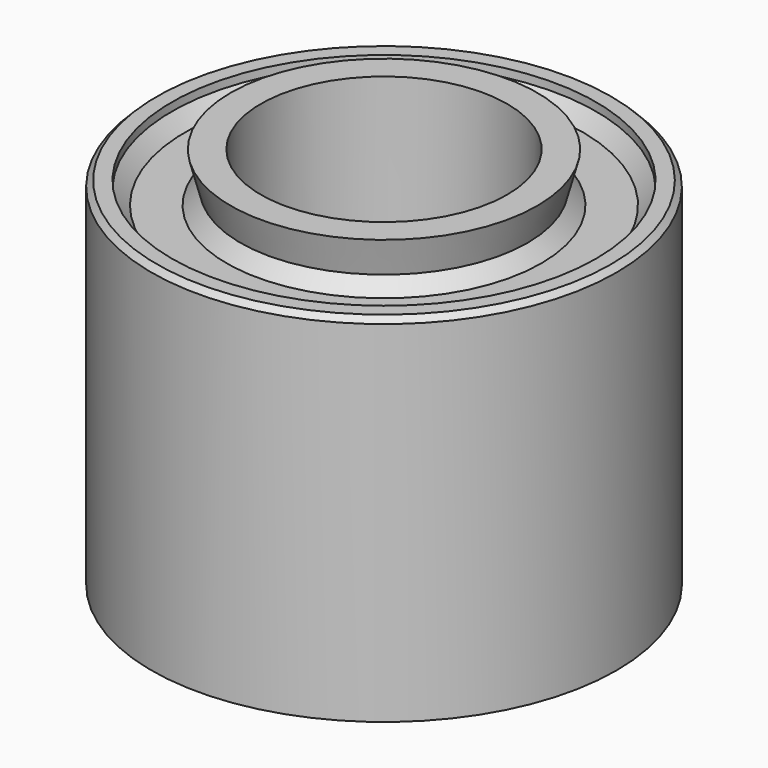
from build123d import *

# Parameters (mm, degrees)
F0_R      = 8.5
F1_DEPTH  = 13
F2_R      = 2.75
F3_DEPTH  = 13.001
F4_R      = 4.5
F5_DEPTH  = 10
F6_SIZE   = 0.2
F7_R      = 7.75
F7_R_2    = 5.25
F8_DEPTH  = 0.8
F9_DEPTH  = 1
F10_R     = 5.6
F10_R_2   = 4.5
F11_DEPTH = 1.5
F11_TAPER = 15


# Not quite as in the source:
# - a fillet or chamfer that OpenCascade refuses, or shapes differently, is made with other operations: its cross-section is extruded or revolved along the edge and cut away or added
# - a feature names something its author has since deleted; it is built from what else it names


with BuildPart() as f1:
    # F0 (on Top) → F1 (new body)
    with BuildSketch(Plane.XY):
        Circle(F0_R)
    extrude(amount=F1_DEPTH)

    # F2 (on face) → F3 (cut, through all)
    with BuildSketch(Plane.XY.offset(13)):
        Circle(F2_R)
    extrude(amount=-F3_DEPTH, mode=Mode.SUBTRACT)

    # F4 (on face) → F5 (cut)
    with BuildSketch(Plane.XY.offset(13)):
        Circle(F4_R)
    extrude(amount=-F5_DEPTH, mode=Mode.SUBTRACT)

    # F6
    f6_edges = [f1.edges().sort_by_distance(p)[0] for p in [
        (-8.5, 0, 13),
    ]]
    chamfer(f6_edges, length=F6_SIZE)

    # F7 (on face) → F8 (cut)
    with BuildSketch(Plane.XY.offset(13)):
        Circle(F7_R)
        Circle(F7_R_2, mode=Mode.SUBTRACT)
    extrude(amount=-F8_DEPTH, mode=Mode.SUBTRACT)

    # F9 (add): a face of the model
    f9_faces = [f1.faces().sort_by_distance(p)[0] for p in [
        (-5.101507576, 0, 13),
    ]]
    extrude(f9_faces, amount=F9_DEPTH)

    # F10 (on face) → F11 (join)
    with BuildSketch(Plane.XY.offset(14)):
        Circle(F10_R)
        Circle(F10_R_2, mode=Mode.SUBTRACT)
    extrude(amount=-F11_DEPTH, taper=F11_TAPER)

    # F12: chamfer of 0.5 on 2 edges, made by hand

    # F12_s1 → F12_t2 (revolve)
    with BuildSketch(Plane.XZ):
        Polygon((7.75, 12.7), (7.25, 12.2), (7.75, 12.2), align=None)
    revolve(axis=Axis((0, 0, 12.2), (0, 0, 1)))

    # F12_s3 → F12_t4 (revolve)
    with BuildSketch(Plane.XZ):
        Polygon((5.75, 12.2), (5.25, 12.7), (5.25, 12.2), align=None)
    revolve(axis=Axis((0, 0, 12.2), (0, 0, 1)))


solid = f1.part
